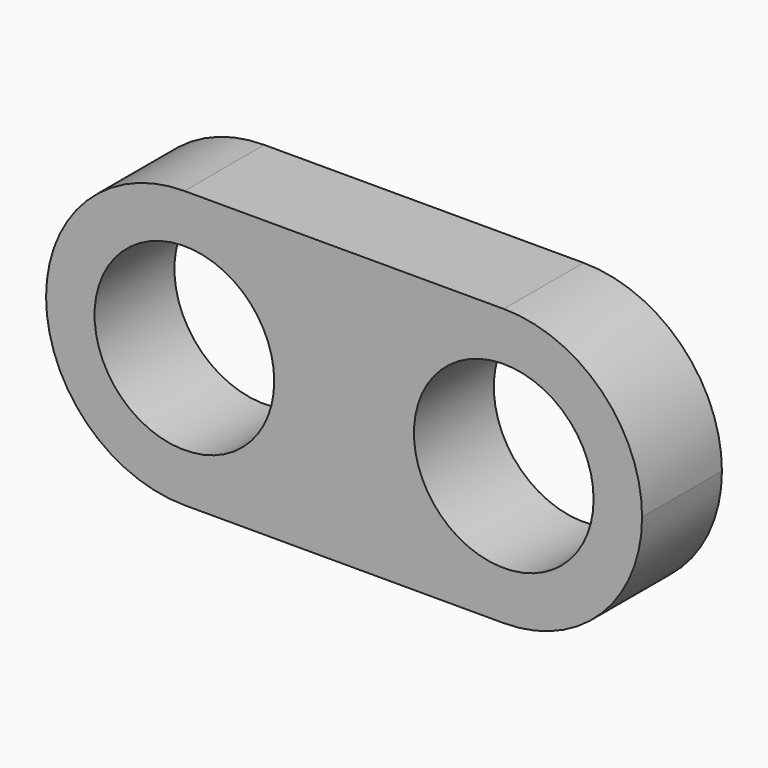
from build123d import *

# Parameters (mm, degrees)
F0_R     = 14.2875
F1_DEPTH = 15.875


# Not quite as in the source:
# - a length typed as a fraction of an inch, garbled in the dataset ("3 / 203.2 mm" for 3/8 in), is restored
# - a feature names something its author has since deleted; it is built from what else it names


with BuildPart() as f1:
    # F0 (on Front) → F1 (new body)
    with BuildSketch(Plane.XZ):
        with BuildLine():
            Line((25.4, 22), (-25.4, 22))
            ThreePointArc((-25.4, 22), (-40.9563491861, 15.5563491861), (-47.4, 0))
            ThreePointArc((-47.4, 0), (-40.9563491861, -15.5563491861), (-25.4, -22))
            Line((-25.4, -22), (25.4, -22))
            ThreePointArc((25.4, -22), (40.9563491861, -15.5563491861), (47.4, 0))
            ThreePointArc((47.4, 0), (40.9563491861, 15.5563491861), (25.4, 22))
        make_face()
        with Locations((-25.4, 0)):
            Circle(F0_R, mode=Mode.SUBTRACT)
        with Locations((25.4, 0)):
            Circle(F0_R, mode=Mode.SUBTRACT)
    extrude(amount=F1_DEPTH)


solid = f1.part
